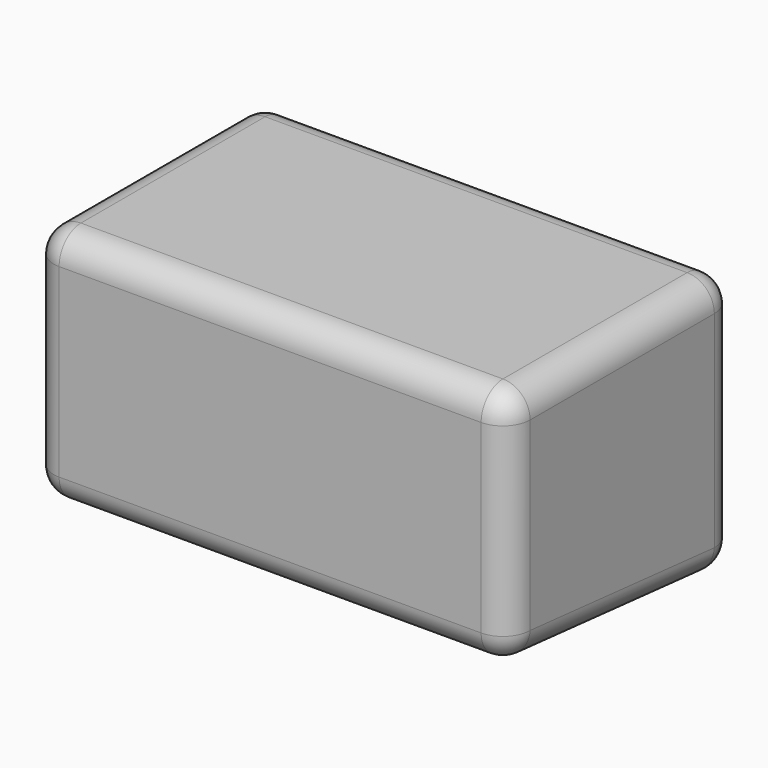
from build123d import *

# Parameters (mm, degrees)
F1_DEPTH = 44.45
F3_R     = 5.08


# Not quite as in the source:
# - a feature of the source that left no trace in its solid (it failed there, or was rolled back) is left out


with BuildPart() as f1:
    # F0 (on Right) → F1 (new body, symmetric)
    with BuildSketch(Plane.YZ):
        Polygon((19.6727830917, 30.9194792062), (-33.4437340498, 30.9194792062), (-33.4437340498, -13.377064839), (19.6727830917, -18.1674808264), align=None)
    extrude(amount=F1_DEPTH, both=True)

    # F3
    f3_edges = [f1.edges().sort_by_distance(p)[0] for p in [
        (-44.45, 19.672783, 6.375999),
        (-44.45, -6.885475, 30.919479),
        (0, -33.443734, 30.919479),
        (44.45, -6.885475, 30.919479),
        (0, 19.672783, 30.919479),
        (44.45, 19.672783, 6.375999),
        (0, 19.672783, -18.167481),
        (0, -33.443734, -13.377065),
        (-44.45, -6.885475, -15.772273),
        (44.45, -6.885475, -15.772273),
        (44.45, -33.443734, 8.771207),
        (-44.45, -33.443734, 8.771207),
    ]]
    fillet(f3_edges, radius=F3_R)


solid = f1.part
